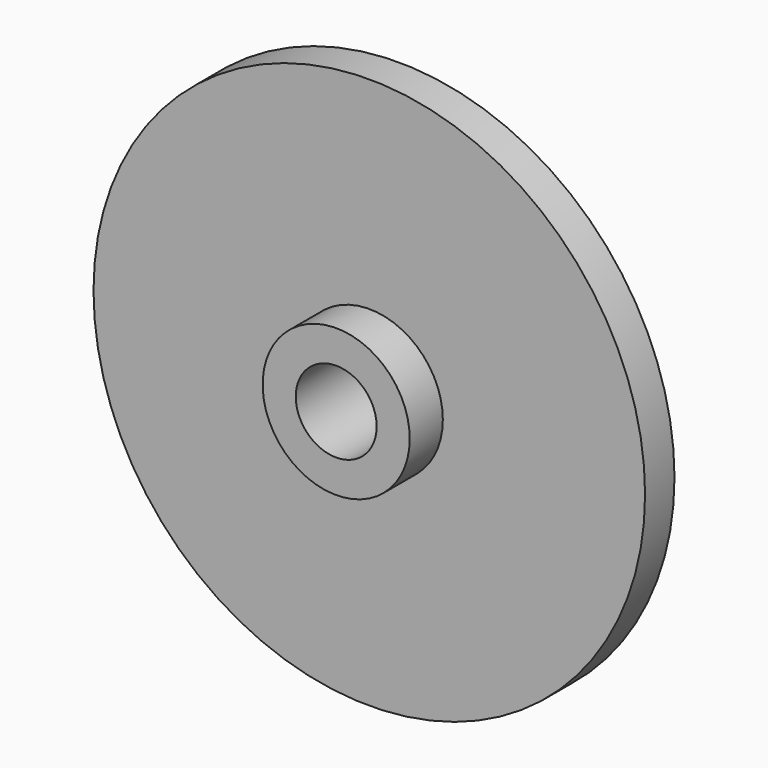
from build123d import *
from build123d import SkipClean  # not in build123d's __all__

# Parameters (mm, degrees)
F0_R     = 15
F1_DEPTH = 2
F2_R     = 4
F3_DEPTH = 2.25
F4_R     = 2.2
F5_DEPTH = 4.251
F6_R     = 4
F6_R_2   = 2.2
F7_DEPTH = 5


with BuildPart() as f1:
    # F0 (on Front) → F1 (new body)
    with BuildSketch(Plane.XZ):
        Circle(F0_R)
    extrude(amount=F1_DEPTH)

    # F2 (on face) → F3 (join)
    with BuildSketch(Plane.XZ.offset(2)):
        Circle(F2_R)
    extrude(amount=F3_DEPTH)

    # F4 (on face) → F5 (cut, through all)
    with BuildSketch(Plane.XZ.offset(4.25)):
        Circle(F4_R)
    extrude(amount=-F5_DEPTH, mode=Mode.SUBTRACT)

    # F6 (on face) → F7 (join)
    with BuildSketch(Plane(origin=(0, 0, 0), x_dir=(-1, 0, 0), z_dir=(0, 1, 0))):
        Circle(F6_R)
        Circle(F6_R_2, mode=Mode.SUBTRACT)
    with SkipClean():  # cleaning this boolean's faces spoils the solid; the shape is the same uncleaned
        extrude(amount=F7_DEPTH)


solid = f1.part
